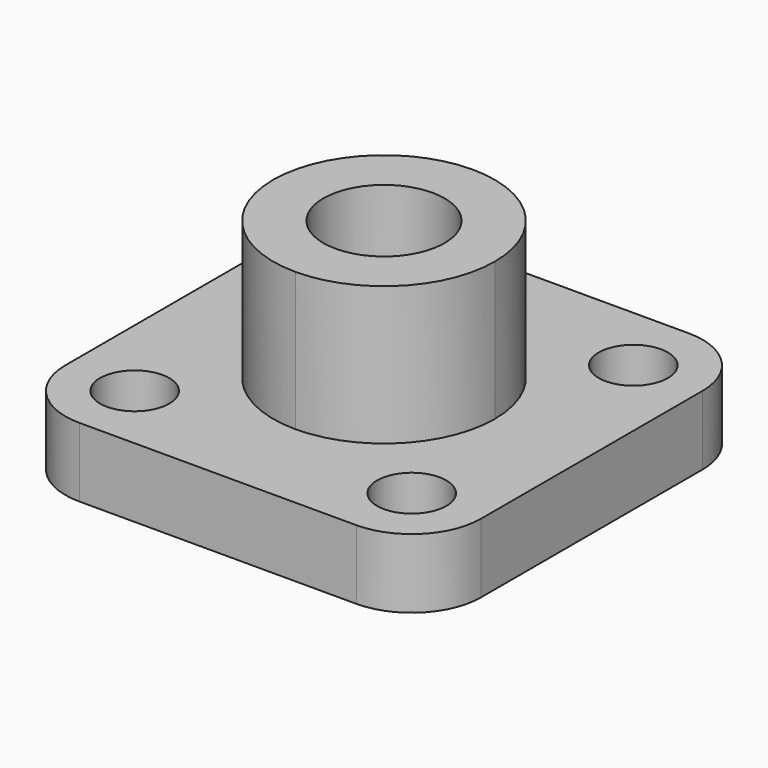
from build123d import *

# Parameters (mm, degrees)
F0_R     = 5
F1_DEPTH = 10
F2_D     = 10
F3_D     = 10
F4_D     = 10
F5_D     = 10
F6_DEPTH = 20
F8_D     = 17.5


with BuildPart() as f1:
    # F0 (on Top) → F1 (new body)
    with BuildSketch(Plane.XY):
        with BuildLine():
            Line((0, 30), (-20, 30))
            ThreePointArc((-20, 30), (-27.0710678119, 27.0710678119), (-30, 20))
            Line((-30, 20), (-30, 0))
            Line((-30, 0), (-16, 0))
            ThreePointArc((-16, 0), (-11.313708499, 11.313708499), (0, 16))
            Line((0, 16), (0, 30))
        make_face()
        with Locations((-20, 20)):
            Circle(F0_R, mode=Mode.SUBTRACT)
        with BuildLine():
            Line((20, 30), (0, 30))
            Line((0, 30), (0, 16))
            ThreePointArc((0, 16), (11.313708499, 11.313708499), (16, 0))
            Line((16, 0), (30, 0))
            Line((30, 0), (30, 20))
            ThreePointArc((30, 20), (27.0710678119, 27.0710678119), (20, 30))
        make_face()
        with Locations((20, 20)):
            Circle(F0_R, mode=Mode.SUBTRACT)
        with BuildLine():
            Line((-16, 0), (-30, 0))
            Line((-30, 0), (-30, -20))
            ThreePointArc((-30, -20), (-27.0710678119, -27.0710678119), (-20, -30))
            Line((-20, -30), (0, -30))
            Line((0, -30), (0, -16))
            ThreePointArc((0, -16), (-11.313708499, -11.313708499), (-16, 0))
        make_face()
        with Locations((-20, -20)):
            Circle(F0_R, mode=Mode.SUBTRACT)
        with BuildLine():
            Line((30, 0), (16, 0))
            ThreePointArc((16, 0), (11.313708499, -11.313708499), (0, -16))
            Line((0, -16), (0, -30))
            Line((0, -30), (20, -30))
            ThreePointArc((20, -30), (27.0710678119, -27.0710678119), (30, -20))
            Line((30, -20), (30, 0))
        make_face()
        with Locations((20, -20)):
            Circle(F0_R, mode=Mode.SUBTRACT)
        with BuildLine():
            Line((0, 0), (0, 16))
            ThreePointArc((0, 16), (-11.313708499, 11.313708499), (-16, 0))
            Line((-16, 0), (0, 0))
        make_face()
        with BuildLine():
            ThreePointArc((16, 0), (11.313708499, 11.313708499), (0, 16))
            Line((0, 16), (0, 0))
            Line((0, 0), (16, 0))
        make_face()
        with BuildLine():
            ThreePointArc((0, -16), (11.313708499, -11.313708499), (16, 0))
            Line((16, 0), (0, 0))
            Line((0, 0), (0, -16))
        make_face()
        with Locations((-20, 20)):
            Circle(F0_R)
        with Locations((20, 20)):
            Circle(F0_R)
        with BuildLine():
            Line((0, 0), (-16, 0))
            ThreePointArc((-16, 0), (-11.313708499, -11.313708499), (0, -16))
            Line((0, -16), (0, 0))
        make_face()
        with Locations((20, -20)):
            Circle(F0_R)
        with Locations((-20, -20)):
            Circle(F0_R)
    extrude(amount=-F1_DEPTH)

    # F2 (through all)
    with Locations(Plane.XY):
        with Locations((-20, 20)):
            Hole(F2_D / 2)

    # F3 (through all)
    with Locations(Plane.XY):
        with Locations((20, 20)):
            Hole(F3_D / 2)

    # F4 (through all)
    with Locations(Plane.XY):
        with Locations((20, -20)):
            Hole(F4_D / 2)

    # F5 (through all)
    with Locations(Plane.XY):
        with Locations((-20, -20)):
            Hole(F5_D / 2)

    # F0 (on Top) → F6 (join)
    with BuildSketch(Plane.XY):
        with BuildLine():
            Line((0, 0), (0, 16))
            ThreePointArc((0, 16), (-11.313708499, 11.313708499), (-16, 0))
            Line((-16, 0), (0, 0))
        make_face()
        with BuildLine():
            ThreePointArc((16, 0), (11.313708499, 11.313708499), (0, 16))
            Line((0, 16), (0, 0))
            Line((0, 0), (16, 0))
        make_face()
        with BuildLine():
            ThreePointArc((0, -16), (11.313708499, -11.313708499), (16, 0))
            Line((16, 0), (0, 0))
            Line((0, 0), (0, -16))
        make_face()
        with BuildLine():
            Line((0, 0), (-16, 0))
            ThreePointArc((-16, 0), (-11.313708499, -11.313708499), (0, -16))
            Line((0, -16), (0, 0))
        make_face()
    extrude(amount=F6_DEPTH)

    # F8 (through all)
    with Locations(Plane.XY.offset(20)):
        with Locations((0, 0)):
            Hole(F8_D / 2)


solid = f1.part
